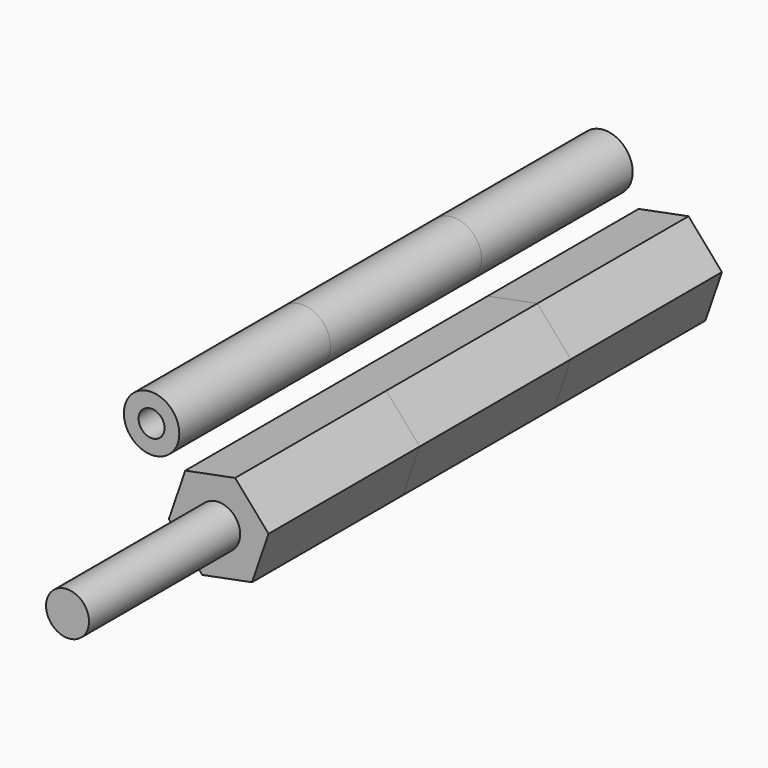
from build123d import *

# Parameters (mm, degrees)
F1_DEPTH = 254
F0_R     = 18.6275130074
F0_R_2   = 8.7223710734
F2_R     = 17.1106148406
F2_R_2   = 18.6275130074
F2_R_3   = 8.7223710734
F3_DEPTH = 127
F4_DEPTH = 127
F6_R     = 14.4488141118
F7_DEPTH = 127


with BuildPart() as f1:
    # F0 (on Front) → F1 (new body)
    with BuildSketch(Plane.XZ):
        Polygon((11.0906781218, 32.3066629883), (-22.4330517984, 25.7581404928), (-33.5237299203, -6.5485224954), (-11.0906781218, -32.3066629883), (22.4330517984, -25.7581404928), (33.5237299203, 6.5485224954), align=None)
    extrude(amount=F1_DEPTH)

    # F2 (on face) + F1_face (on face) → F3 (join)
    with BuildSketch(Plane.XZ.offset(254)):
        Circle(F2_R)
        with Locations((-45.0995638967, 46.2823174894)):
            Circle(F2_R_2)
        with Locations((-45.0995638967, 46.2823174894)):
            Circle(F2_R_3, mode=Mode.SUBTRACT)
    with BuildSketch(Plane(origin=(-45.0995638967, -254, 46.2823174894), x_dir=(1, 0, 0), z_dir=(0, -1, 0))):
        Polygon((56.1902420185, -13.9756545011), (22.6665120982, -20.5241769966), (11.5758339764, -52.8308399848), (34.0088857748, -78.5889804777), (67.5326156951, -72.0404579822), (78.6232938169, -39.733794994), align=None)
    extrude(amount=F3_DEPTH)


with BuildPart() as f1b:
    # F0 (on Front) → F1, piece 2 (new body)
    with BuildSketch(Plane.XZ):
        with Locations((-45.0995638967, 46.2823174894)):
            Circle(F0_R)
        with Locations((-45.0995638967, 46.2823174894)):
            Circle(F0_R_2, mode=Mode.SUBTRACT)
    extrude(amount=F1_DEPTH)


with BuildPart() as f4:
    # F0 (on Front) → F4 (new body)
    with BuildSketch(Plane.XZ):
        Polygon((11.0906781218, 32.3066629883), (-22.4330517984, 25.7581404928), (-33.5237299203, -6.5485224954), (-11.0906781218, -32.3066629883), (22.4330517984, -25.7581404928), (33.5237299203, 6.5485224954), align=None)
    extrude(amount=F4_DEPTH)


with BuildPart() as f4b:
    # F0 (on Front) → F4, piece 2 (new body)
    with BuildSketch(Plane.XZ):
        with Locations((-45.0995638967, 46.2823174894)):
            Circle(F0_R)
        with Locations((-45.0995638967, 46.2823174894)):
            Circle(F0_R_2, mode=Mode.SUBTRACT)
    extrude(amount=F4_DEPTH)


with BuildPart() as f7:
    # F6 (on face) + F1_face1 (on face) → F7 (new body)
    with BuildSketch(Plane.XZ.offset(381)):
        Circle(F6_R)
    with BuildSketch(Plane(origin=(0, 0, 0), x_dir=(1, 0, 0), z_dir=(0, 1, 0))):
        Polygon((-22.4330517984, -25.7581404928), (11.0906781218, -32.3066629883), (33.5237299203, -6.5485224954), (22.4330517984, 25.7581404928), (-11.0906781218, 32.3066629883), (-33.5237299203, 6.5485224954), align=None)
    extrude(amount=F7_DEPTH, dir=(0, -1, 0))


solid = Compound([f1.part, f1b.part, f4.part, f4b.part, f7.part])
